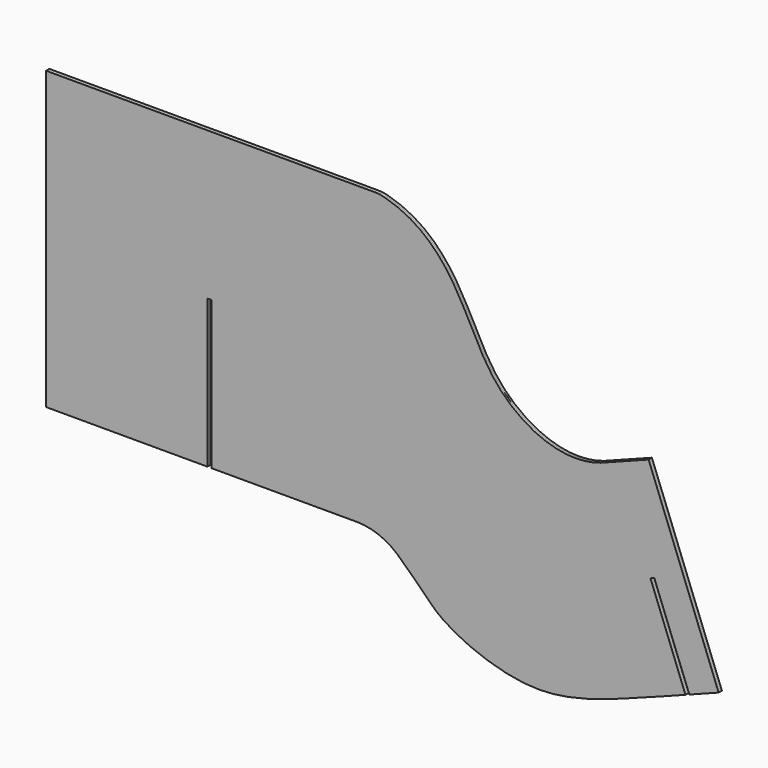
from build123d import *

# Parameters (mm, degrees)
F1_DEPTH = 1


with BuildPart() as f1:
    # F0 (on Front) → F1 (new body, symmetric)
    with BuildSketch(Plane.XZ):
        with BuildLine():
            Line((78.5832557587, 72), (-81, 72))
            Line((-81, 72), (-81, -72))
            Line((-81, -72), (-2.5758354459, -72))
            Line((-2.5758354459, -72), (-2.5758354459, 0))
            Line((-2.5758354459, 0), (-0.5758354459, 0))
            Line((-0.5758354459, 0), (-0.5758354459, -72))
            Line((-0.5758354459, -72), (70.0140722752, -72))
            ThreePointArc((70.0140722752, -72), (80.6669131732, -73.9550899306), (89.9312699398, -79.5655346133))
            add(Edge.make_bspline(
                [(81, -72), (84.4635983749, -74.8141629135), (87.3994420895, -77.31779147), (89.9312699398, -79.5655346133)],
                knots=[0, 0, 0, 0, 0.0519635784, 0.0519635784, 0.0519635784, 0.0519635784], degree=3))
            Line((81, -72), (81, 71.8534467353))
            ThreePointArc((81, 71.8534467353), (79.7938476168, 71.9633280631), (78.5832557587, 72))
        make_face()
        with BuildLine():
            Line((81, 72), (81, 71.8534467353))
            Line((81, 71.8534467353), (81, -72))
            add(Edge.make_bspline(
                [(81, -72), (84.4635983749, -74.8141629135), (87.3994420895, -77.31779147), (89.9312699398, -79.5655346133)],
                knots=[0, 0, 0, 0, 0.0519635784, 0.0519635784, 0.0519635784, 0.0519635784], degree=3))
            add(Edge.make_bspline(
                [(89.9312699398, -79.5655346133), (102.3651827748, -90.6042955291), (108.3217609729, -101.383114475), (158.7265599507, -121.9444495797), (190.0937696642, -109.2006741806), (218.0848423474, -98.6219057368)],
                knots=[0.0519635784, 0.0519635784, 0.0519635784, 0.0519635784, 0.3071588928, 0.6171111846, 1, 1, 1, 1], degree=3))
            Line((218.0848423474, -98.6219057368), (229.9621609222, -94.0626303033))
            Line((229.9621609222, -94.0626303033), (212.9396833188, -49.7175600446))
            Line((212.9396833188, -49.7175600446), (214.8068441718, -49.0008241456))
            Line((214.8068441718, -49.0008241456), (231.8293217752, -93.3458944042))
            Line((231.8293217752, -93.3458944042), (246.0922551423, -87.8708672505))
            Line((246.0922551423, -87.8708672505), (212.0472999355, 0.8192732668))
            Line((212.0472999355, 0.8192732668), (188.707789273, -8.1399254719))
            add(Edge.make_bspline(
                [(83.8849046159, 71.2845150158), (105.3400246798, 65.3861290478), (124.0549392531, 35.6814961762), (138.1532322102, 1.7025226497), (170.7937318796, -14.1268512491), (188.707789273, -8.1399254719)],
                knots=[0.0153089318, 0.0153089318, 0.0153089318, 0.0153089318, 0.3648606153, 0.6619581151, 1, 1, 1, 1], degree=3))
            add(Edge.make_bspline(
                [(81, 72), (81.9838635002, 71.7816800805), (82.9452582497, 71.542840158), (83.8849046159, 71.2845150158)],
                knots=[0, 0, 0, 0, 0.0153089318, 0.0153089318, 0.0153089318, 0.0153089318], degree=3))
        make_face()
        with BuildLine():
            ThreePointArc((83.8849046159, 71.2845150158), (82.45292226, 71.6220712762), (81, 71.8534467353))
            Line((81, 71.8534467353), (81, 72))
            add(Edge.make_bspline(
                [(81, 72), (81.9838635002, 71.7816800805), (82.9452582497, 71.542840158), (83.8849046159, 71.2845150158)],
                knots=[0, 0, 0, 0, 0.0153089318, 0.0153089318, 0.0153089318, 0.0153089318], degree=3))
        make_face(mode=Mode.SUBTRACT)
    extrude(amount=F1_DEPTH, both=True)


solid = f1.part
